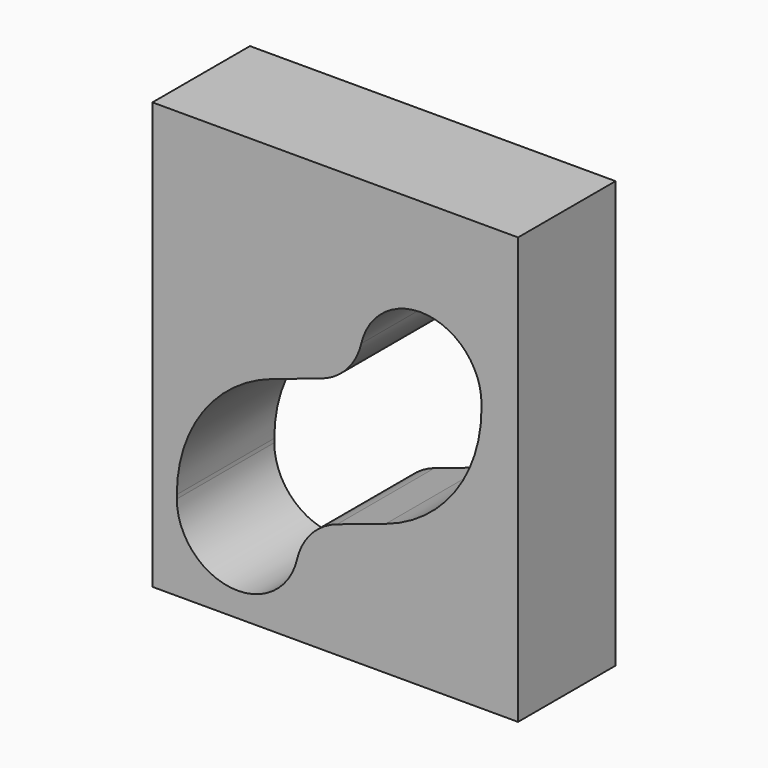
from build123d import *

# Parameters (mm, degrees)
F0_W     = 30
F0_H     = 35
F1_DEPTH = 10
F3_DEPTH = 10.001


# Not quite as in the source:
# - ends of sketch curves that miss each other by under 0.0002 mm in the source are joined


with BuildPart() as f1:
    # F0 (on Front) → F1 (new body)
    with BuildSketch(Plane.XZ):
        with Locations((15, 17.5)):
            Rectangle(F0_W, F0_H)
    extrude(amount=F1_DEPTH)

    # F2 (on face) → F3 (cut, through all)
    with BuildSketch(Plane.XZ.offset(10)):
        with BuildLine():
            Line((2.000000095, 7.3150651013), (2.000000095, 7))
            ThreePointArc((2.000000095, 7), (6.4219498037, 2.0335266063), (11.8663431882, 5.8516516319))
            ThreePointArc((11.8663431882, 5.8516516319), (13.0416655427, 8.0761900401), (15.1515475464, 9.4467197541))
            Line((15.1515475464, 9.4467197541), (19.1366200095, 10.7750772419))
            ThreePointArc((19.1366200095, 10.7750772419), (24.8292858299, 14.9607668958), (27.0000007004, 21.6849351694))
            Line((27.0000007004, 21.6849351694), (27.0000007004, 22))
            ThreePointArc((27.0000007004, 22), (22.5780501979, 26.9664733935), (17.1336568125, 23.1483483711))
            ThreePointArc((17.1336568125, 23.1483483711), (15.9583344576, 20.9238099649), (13.8484524551, 19.553280252))
            Line((13.8484524551, 19.553280252), (9.8633807858, 18.2249230289))
            ThreePointArc((9.8633807858, 18.2249230289), (4.1707149655, 14.0392333749), (2.000000095, 7.3150651013))
        make_face()
    extrude(amount=-F3_DEPTH, mode=Mode.SUBTRACT)


solid = f1.part
